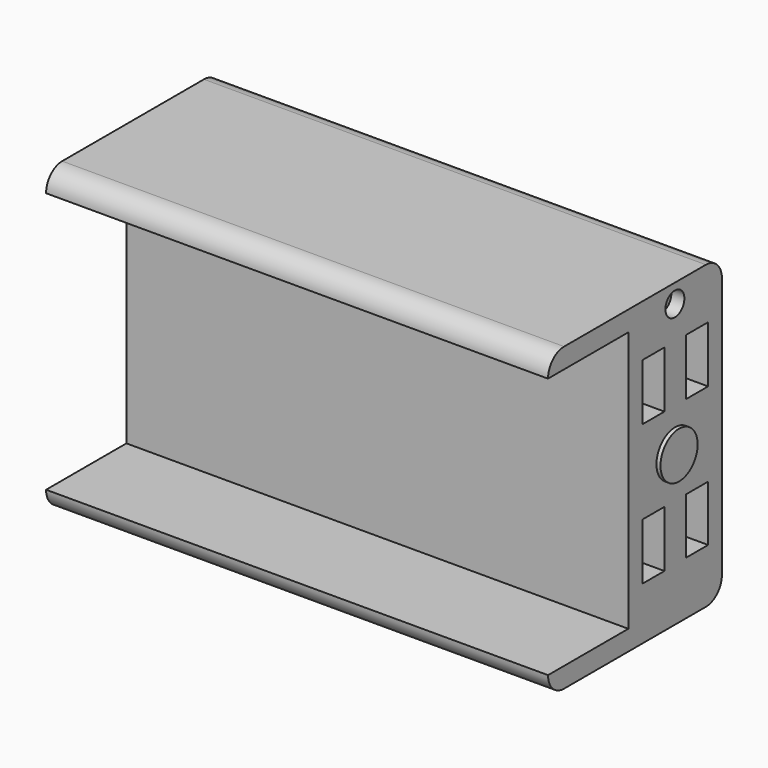
from build123d import *

# Parameters (mm, degrees)
F0_W         = 127
F0_H         = 76.2
F1_DEPTH     = 55
F2_R         = 5.08
F3_W         = 7
F3_H         = 14.3
F4_DEPTH     = 16.4
F5_DEPTH     = 25.4
F6_W         = 7
F6_H         = 14.3
F6_W_2       = 7.0104
F6_H_2       = 14.117781591
F7_DEPTH     = 16.4
F9_W         = 19.8135651034
F9_H         = 65.8797910702
F10_DEPTH    = 2.54
F11_T1_DEPTH = 87.8768363263
F11_T3_DEPTH = 41.8106103595
F12_DEPTH    = 1.524
F13_R        = 3
F13_R_2      = 1.8
F14_DEPTH    = 3.3
F15_DEPTH    = 11
F8_R         = 5.878920021
F16_DEPTH    = 1.016


# Not quite as in the source:
# - a fillet or chamfer that OpenCascade refuses, or shapes differently, is made with other operations: its cross-section is extruded or revolved along the edge and cut away or added


with BuildPart() as f1:
    # F0 (on Front) → F1 (new body)
    with BuildSketch(Plane.XZ):
        Rectangle(F0_W, F0_H)
    extrude(amount=F1_DEPTH)

    # F2
    f2_edges = [f1.edges().sort_by_distance(p)[0] for p in [
        (0, -55, -38.1),
        (0, 0, -38.1),
        (0, -55, 38.1),
        (0, 0, 38.1),
    ]]
    fillet(f2_edges, radius=F2_R)

    # F3 (on face) → F4 (cut)
    with BuildSketch(Plane.YZ.offset(63.5)):
        with Locations((-49.3123565018, 17.8676303864)):
            Rectangle(F3_W, F3_H)
        with Locations((-35.2098751962, 17.8676303864)):
            Rectangle(F3_W, F3_H)
        with Locations((-21.6830033958, 17.8676303864)):
            Rectangle(F3_W, F3_H)
        with Locations((-7.8683277741, 17.8676303864)):
            Rectangle(F3_W, F3_H)
    extrude(amount=-F4_DEPTH, mode=Mode.SUBTRACT)

    # F5 (cut): a face of the model
    f5_faces = [f1.faces().sort_by_distance(p)[0] for p in [
        (0, -55, 0),
    ]]
    extrude(f5_faces, amount=-F5_DEPTH, mode=Mode.SUBTRACT)

    # F6 (on face) → F7 (cut)
    with BuildSketch(Plane.YZ.offset(63.5)):
        with Locations((-21.6830033958, -17.639610437)):
            Rectangle(F6_W, F6_H)
        with Locations((-7.8631268428, -17.5485012325)):
            Rectangle(F6_W_2, F6_H_2)
    extrude(amount=-F7_DEPTH, mode=Mode.SUBTRACT)

    # F9 (on face) → F10 (join)
    with BuildSketch(Plane(origin=(-63.5, 0, 0), x_dir=(0, -1, 0), z_dir=(-1, 0, 0))):
        with Locations((14.9867825517, 0.0801044649)):
            Rectangle(F9_W, F9_H)
    extrude(amount=F10_DEPTH)

    # F11: fillet of radius 5.08 on 4 edges, made by hand

    # F11_s2 → F11_t1 (cut)
    with BuildSketch(Plane.XY.offset(-43.8583136983)):
        with BuildLine():
            ThreePointArc((-63.5, -24.8935651034), (-65.3594090512, -23.0341560522), (-66.04, -20.4941560522))
            Line((-66.04, -20.4941560522), (-66.04, -24.8935651034))
            Line((-66.04, -24.8935651034), (-63.5, -24.8935651034))
        make_face()
        with BuildLine():
            ThreePointArc((-63.5, -5.08), (-65.3594090512, -6.9394090512), (-66.04, -9.4794090512))
            Line((-66.04, -9.4794090512), (-66.04, -5.08))
            Line((-66.04, -5.08), (-63.5, -5.08))
        make_face()
    extrude(amount=F11_T1_DEPTH, mode=Mode.SUBTRACT)

    # F11_s4 → F11_t3 (cut)
    with BuildSketch(Plane.XZ.offset(-5.9185226281)):
        with BuildLine():
            ThreePointArc((-63.5, 33.02), (-65.3594090512, 31.1605909488), (-66.04, 28.6205909488))
            Line((-66.04, 28.6205909488), (-66.04, 33.02))
            Line((-66.04, 33.02), (-63.5, 33.02))
        make_face()
        with BuildLine():
            ThreePointArc((-63.5, -32.8597910702), (-65.3594090512, -31.000382019), (-66.04, -28.460382019))
            Line((-66.04, -28.460382019), (-66.04, -32.8597910702))
            Line((-66.04, -32.8597910702), (-63.5, -32.8597910702))
        make_face()
    extrude(amount=F11_T3_DEPTH, mode=Mode.SUBTRACT)

    # F12 (cut): a face of the model
    f12_faces = [f1.faces().sort_by_distance(p)[0] for p in [
        (-66.04, -14.9867825517, 0.0801044649),
    ]]
    extrude(f12_faces, amount=-F12_DEPTH, mode=Mode.SUBTRACT)

    # F13 (on face) → F14 (cut)
    with BuildSketch(Plane.YZ.offset(63.5)):
        with Locations((-14.8709248751, 33.3571620286)):
            Circle(F13_R)
        with Locations((-14.8709248751, 33.3571620286)):
            Circle(F13_R_2, mode=Mode.SUBTRACT)
    extrude(amount=-F14_DEPTH, mode=Mode.SUBTRACT)

    # F15 (cut): a face of the model
    f15_faces = [f1.faces().sort_by_distance(p)[0] for p in [
        (63.5, -14.8709248751, 33.3571620286),
    ]]
    extrude(f15_faces, amount=-F15_DEPTH, mode=Mode.SUBTRACT)

    # F8 (on face) → F16 (join)
    with BuildSketch(Plane.YZ.offset(63.5)):
        with Locations((-14.821995981, 0)):
            Circle(F8_R)
    extrude(amount=F16_DEPTH)


solid = f1.part
